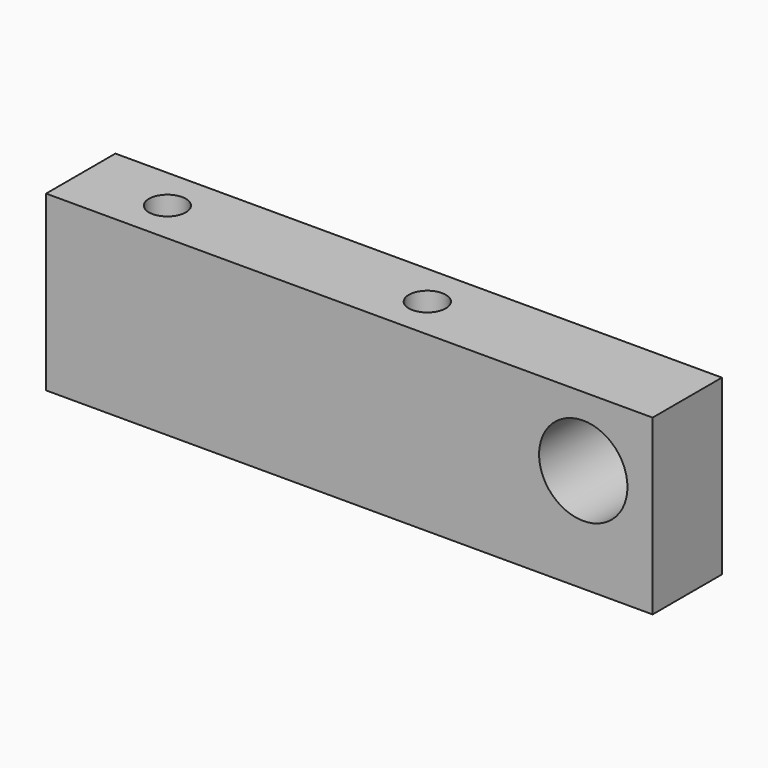
from build123d import *

# Parameters (mm, degrees)
F0_W     = 44.45
F0_H     = 12.7
F0_R     = 3.2385
F1_DEPTH = 6.35
F3_D     = 2.7051


with BuildPart() as f1:
    # F0 (on Front) → F1 (new body)
    with BuildSketch(Plane.XZ):
        Rectangle(F0_W, F0_H)
        with Locations((17.145, 1.27)):
            Circle(F0_R, mode=Mode.SUBTRACT)
    extrude(amount=F1_DEPTH)

    # F3 (through all)
    with Locations(Plane(origin=(0, 0, -6.35), x_dir=(1, 0, 0), z_dir=(0, 0, -1))):
        with Locations((-15.875, 3.175), (3.175, 3.175)):
            Hole(F3_D / 2)


solid = f1.part
